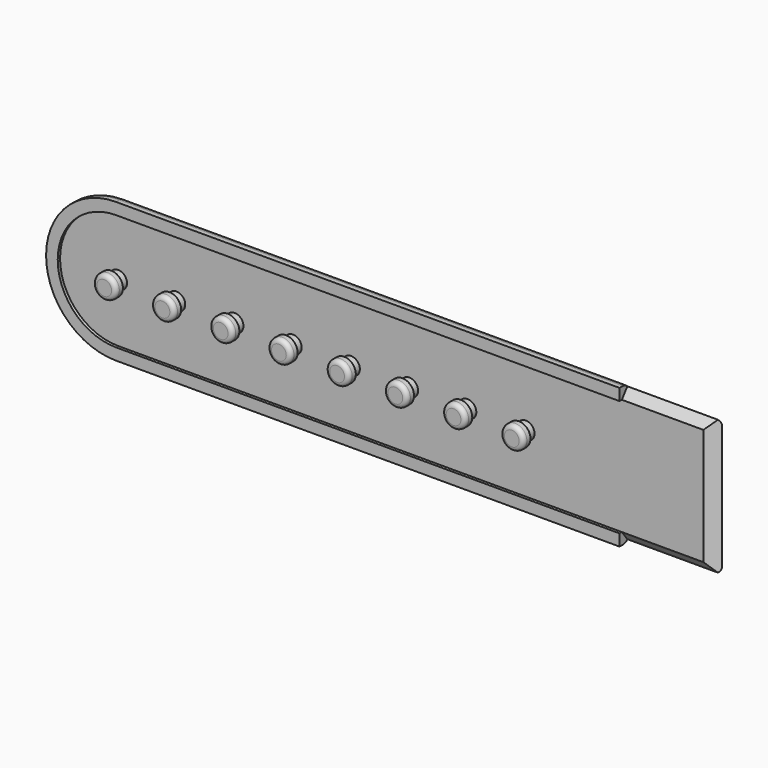
from build123d import *

# Parameters (mm, degrees)
F1_DEPTH     = 1.5875
F0_R         = 1.5875
F0_R_2       = 1.190625
F2_DEPTH     = 1.18872
F3_DEPTH     = 1.18872
F4_T1_DEPTH  = 27.2432951274
F4_T6_DEPTH  = 16.7966475637
F4_T11_DEPTH = 16.7966475637
F5_DEPTH     = 3.5814
F6_START     = 2.37744
F6_DEPTH     = 1.20396
F7_R         = 0.5842
F8_R         = 1.016


# Not quite as in the source:
# - a fillet or chamfer that OpenCascade refuses, or shapes differently, is made with other operations: its cross-section is extruded or revolved along the edge and cut away or added


with BuildPart() as f1:
    # F0 (on Front) → F1 (new body)
    with BuildSketch(Plane.XZ):
        with BuildLine():
            Line((-81.3593362805, 0), (-12.7, 0))
            Line((-12.7, 0), (-12.7, 1.5875))
            Line((-12.7, 1.5875), (-81.3593362805, 1.5875))
            ThreePointArc((-81.3593362805, 1.5875), (-89.2968362805, 9.525), (-81.3593362805, 17.4625))
            Line((-81.3593362805, 17.4625), (-12.7, 17.4625))
            Line((-12.7, 17.4625), (-12.7, 19.05))
            Line((-12.7, 19.05), (-81.3593362805, 19.05))
            ThreePointArc((-81.3593362805, 19.05), (-90.8843362805, 9.525), (-81.3593362805, 0))
        make_face()
    extrude(amount=F1_DEPTH)

    # F0 (on Front) → F2 (join)
    with BuildSketch(Plane.XZ):
        with BuildLine():
            Line((-81.3593362805, 1.5875), (-12.7, 1.5875))
            Line((-12.7, 1.5875), (-1.5875, 1.5875))
            Line((-1.5875, 1.5875), (-1.5875, 17.4625))
            Line((-1.5875, 17.4625), (-12.7, 17.4625))
            Line((-12.7, 17.4625), (-81.3593362805, 17.4625))
            ThreePointArc((-81.3593362805, 17.4625), (-89.2968362805, 9.525), (-81.3593362805, 1.5875))
        make_face()
        with Locations((-81.3593362805, 9.525)):
            Circle(F0_R, mode=Mode.SUBTRACT)
        with Locations((-73.4218362805, 9.525)):
            Circle(F0_R, mode=Mode.SUBTRACT)
        with Locations((-65.4843362805, 9.525)):
            Circle(F0_R, mode=Mode.SUBTRACT)
        with Locations((-57.5468362805, 9.525)):
            Circle(F0_R, mode=Mode.SUBTRACT)
        with Locations((-49.6093362805, 9.525)):
            Circle(F0_R, mode=Mode.SUBTRACT)
        with Locations((-41.6718362805, 9.525)):
            Circle(F0_R, mode=Mode.SUBTRACT)
        with Locations((-33.7343362805, 9.525)):
            Circle(F0_R, mode=Mode.SUBTRACT)
        with Locations((-25.7968362805, 9.525)):
            Circle(F0_R, mode=Mode.SUBTRACT)
        with Locations((-81.3593362805, 9.525)):
            Circle(F0_R)
        with Locations((-81.3593362805, 9.525)):
            Circle(F0_R_2, mode=Mode.SUBTRACT)
        with Locations((-73.4218362805, 9.525)):
            Circle(F0_R)
        with Locations((-73.4218362805, 9.525)):
            Circle(F0_R_2, mode=Mode.SUBTRACT)
        with Locations((-65.4843362805, 9.525)):
            Circle(F0_R)
        with Locations((-65.4843362805, 9.525)):
            Circle(F0_R_2, mode=Mode.SUBTRACT)
        with Locations((-57.5468362805, 9.525)):
            Circle(F0_R)
        with Locations((-57.5468362805, 9.525)):
            Circle(F0_R_2, mode=Mode.SUBTRACT)
        with Locations((-49.6093362805, 9.525)):
            Circle(F0_R)
        with Locations((-49.6093362805, 9.525)):
            Circle(F0_R_2, mode=Mode.SUBTRACT)
        with Locations((-41.6718362805, 9.525)):
            Circle(F0_R)
        with Locations((-41.6718362805, 9.525)):
            Circle(F0_R_2, mode=Mode.SUBTRACT)
        with Locations((-33.7343362805, 9.525)):
            Circle(F0_R)
        with Locations((-33.7343362805, 9.525)):
            Circle(F0_R_2, mode=Mode.SUBTRACT)
        with Locations((-25.7968362805, 9.525)):
            Circle(F0_R)
        with Locations((-25.7968362805, 9.525)):
            Circle(F0_R_2, mode=Mode.SUBTRACT)
    extrude(amount=F2_DEPTH)

    # F0 (on Front) → F3 (join)
    with BuildSketch(Plane.XZ):
        Polygon((-12.7, 0), (0, 0), (0, 19.05), (-12.7, 19.05), (-12.7, 17.4625), (-1.5875, 17.4625), (-1.5875, 1.5875), (-12.7, 1.5875), align=None)
    extrude(amount=F3_DEPTH)

    # F4: chamfer of 1.5875 x 1.1962670545 on 3 edges, made by hand

    # F4_s2 → F4_t1 (cut)
    with BuildSketch(Plane.XY.offset(-4.0966475637)):
        Polygon((-1.5875, -1.18872), (0, 0.0075470545), (0, -1.18872), align=None)
    extrude(amount=F4_T1_DEPTH, mode=Mode.SUBTRACT)


with BuildPart() as f4_tool4:
    # F4_s5 → F4_t6 (new body)
    with BuildSketch(Plane.YZ.offset(4.0966475637)):
        Polygon((-1.18872, 17.4625), (0.0075470545, 19.05), (-1.18872, 19.05), align=None)
    extrude(amount=-F4_T6_DEPTH)

    split(bisect_by=Plane.XY.offset(17.4625), keep=Keep.TOP)


with BuildPart() as f1_1:
    add(f1.part)

    # F4_t3: cut F4_tool4
    add(f4_tool4.part, mode=Mode.SUBTRACT)


with BuildPart() as f4_tool9:
    # F4_s10 → F4_t11 (new body)
    with BuildSketch(Plane.YZ.offset(-12.7)):
        Polygon((-1.18872, 1.5875), (0.0075470545, 0), (-1.18872, 0), align=None)
    extrude(amount=F4_T11_DEPTH)

    split(bisect_by=Plane.XY.offset(1.5875), keep=Keep.BOTTOM)


with BuildPart() as f1_2:
    add(f1_1.part)

    # F4_t8: cut F4_tool9
    add(f4_tool9.part, mode=Mode.SUBTRACT)

    # F0 (on Front) → F5 (join)
    with BuildSketch(Plane.XZ):
        with Locations((-81.3593362805, 9.525)):
            Circle(F0_R_2)
        with Locations((-73.4218362805, 9.525)):
            Circle(F0_R_2)
        with Locations((-65.4843362805, 9.525)):
            Circle(F0_R_2)
        with Locations((-57.5468362805, 9.525)):
            Circle(F0_R_2)
        with Locations((-49.6093362805, 9.525)):
            Circle(F0_R_2)
        with Locations((-41.6718362805, 9.525)):
            Circle(F0_R_2)
        with Locations((-33.7343362805, 9.525)):
            Circle(F0_R_2)
        with Locations((-25.7968362805, 9.525)):
            Circle(F0_R_2)
    extrude(amount=F5_DEPTH)

    # F0 (on Front) → F6 (join)
    with BuildSketch(Plane.XZ.offset(F6_START)):
        with Locations((-81.3593362805, 9.525)):
            Circle(F0_R)
        with Locations((-81.3593362805, 9.525)):
            Circle(F0_R_2, mode=Mode.SUBTRACT)
        with Locations((-73.4218362805, 9.525)):
            Circle(F0_R)
        with Locations((-73.4218362805, 9.525)):
            Circle(F0_R_2, mode=Mode.SUBTRACT)
        with Locations((-65.4843362805, 9.525)):
            Circle(F0_R)
        with Locations((-65.4843362805, 9.525)):
            Circle(F0_R_2, mode=Mode.SUBTRACT)
        with Locations((-57.5468362805, 9.525)):
            Circle(F0_R)
        with Locations((-57.5468362805, 9.525)):
            Circle(F0_R_2, mode=Mode.SUBTRACT)
        with Locations((-49.6093362805, 9.525)):
            Circle(F0_R)
        with Locations((-49.6093362805, 9.525)):
            Circle(F0_R_2, mode=Mode.SUBTRACT)
        with Locations((-41.6718362805, 9.525)):
            Circle(F0_R)
        with Locations((-41.6718362805, 9.525)):
            Circle(F0_R_2, mode=Mode.SUBTRACT)
        with Locations((-33.7343362805, 9.525)):
            Circle(F0_R)
        with Locations((-33.7343362805, 9.525)):
            Circle(F0_R_2, mode=Mode.SUBTRACT)
        with Locations((-25.7968362805, 9.525)):
            Circle(F0_R)
        with Locations((-25.7968362805, 9.525)):
            Circle(F0_R_2, mode=Mode.SUBTRACT)
    extrude(amount=F6_DEPTH)

    # F7
    f7_edges = [f1_2.edges().sort_by_distance(p)[0] for p in [
        (-82.946836, -3.5814, 9.525),
        (-75.009336, -3.5814, 9.525),
        (-67.071836, -3.5814, 9.525),
        (-59.134336, -3.5814, 9.525),
        (-51.196836, -3.5814, 9.525),
        (-43.259336, -3.5814, 9.525),
        (-35.321836, -3.5814, 9.525),
        (-27.384336, -3.5814, 9.525),
    ]]
    fillet(f7_edges, radius=F7_R)

    # F8
    f8_edges = [f1_2.edges().sort_by_distance(p)[0] for p in [
        (-47.029668, 0, 0),
        (-90.884336, 0, 9.525),
        (-47.029668, 0, 19.05),
    ]]
    fillet(f8_edges, radius=F8_R)


solid = f1_2.part
